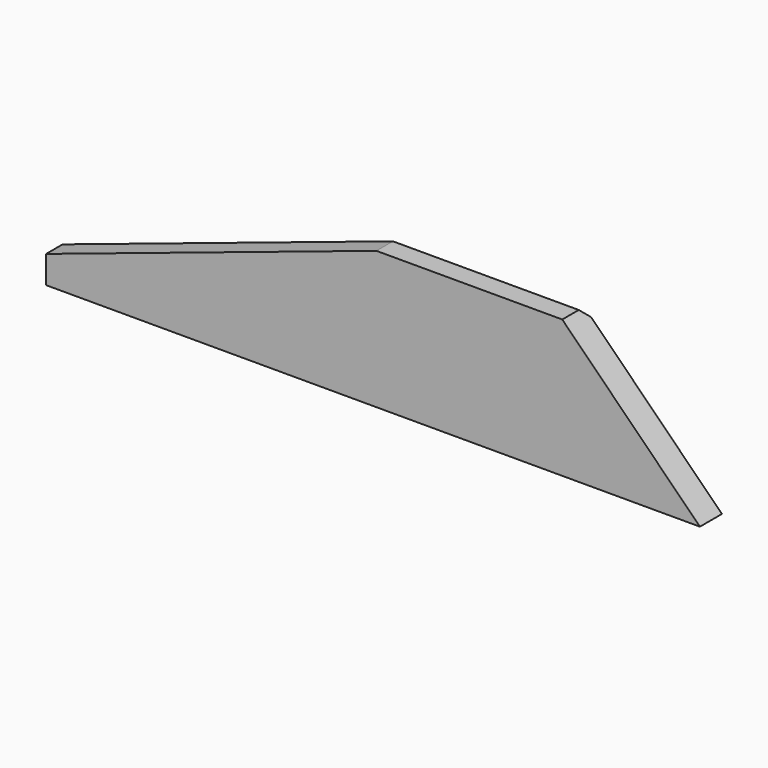
from build123d import *

# Parameters (mm, degrees)
F1_DEPTH = 20
F2_SIZE  = 5
F3_SIZE  = 99.99999


# Not quite as in the source:
# - a fillet or chamfer is up to 0.001 mm smaller than in the source, because OpenCascade refuses the exact size


with BuildPart() as f1:
    # F0 (on Front) → F1 (new body)
    with BuildSketch(Plane.XZ):
        Polygon((-227.9723286629, -18.1198753417), (247.0276713371, -18.1198753417), (247.0276713371, 81.8801246583), (12.0276713371, 81.8801246583), (-227.9723286629, 1.8801246583), align=None)
    extrude(amount=F1_DEPTH)

    # F2
    f2_edges = [f1.edges().sort_by_distance(p)[0] for p in [
        (129.527671, 0, 81.880125),
        (-107.972329, 0, 41.880125),
        (-227.972329, 0, -8.119875),
    ]]
    chamfer(f2_edges, length=F2_SIZE)

    # F3 (size 100 in the source; OpenCascade refuses exactly that, so slightly less here)
    f3_edges = [f1.edges().sort_by_distance(p)[0] for p in [
        (247.027671, -12.5, 81.880125),
    ]]
    chamfer(f3_edges, length=F3_SIZE)


solid = f1.part
